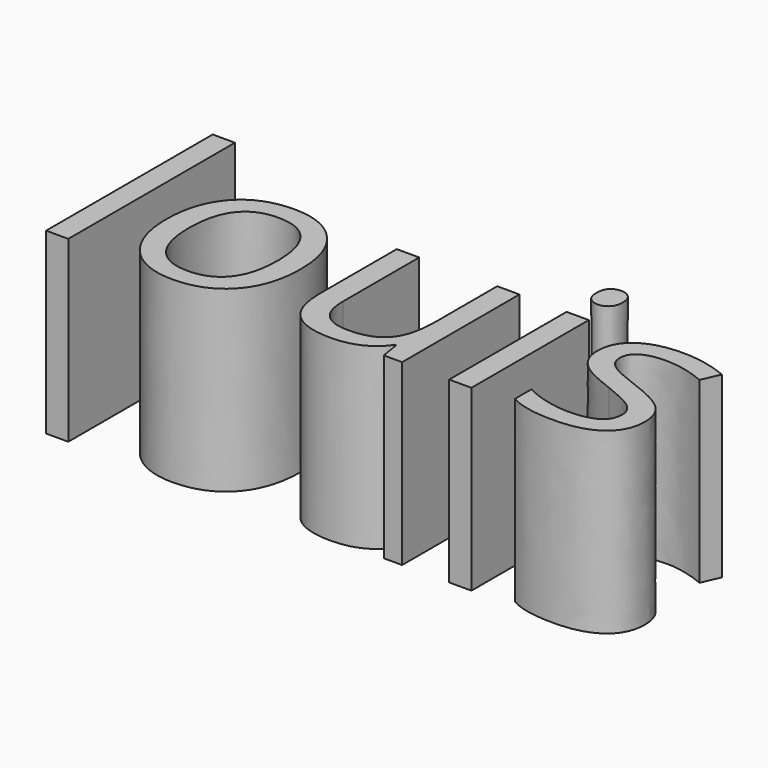
from build123d import *

# Parameters (mm, degrees)
F0_TEXT_SIZE = 76.7257530242
F1_DEPTH     = 50


# Not quite as in the source:
# - Text() gives the source's letters only with a copy of the font that has no kerning and outlines rounded to 1/6400 em; it was checked with that copy


with BuildPart() as f1:
    # F0 (on Top) → F1 (new body)
    with BuildSketch(Plane.XY):
        with Locations((-170.3071949159, -55.2425421774)):
            Text('louis', F0_TEXT_SIZE, font='Open Sans', text_align=(TextAlign.LEFT, TextAlign.BOTTOM))
    extrude(amount=F1_DEPTH)


solid = f1.part
